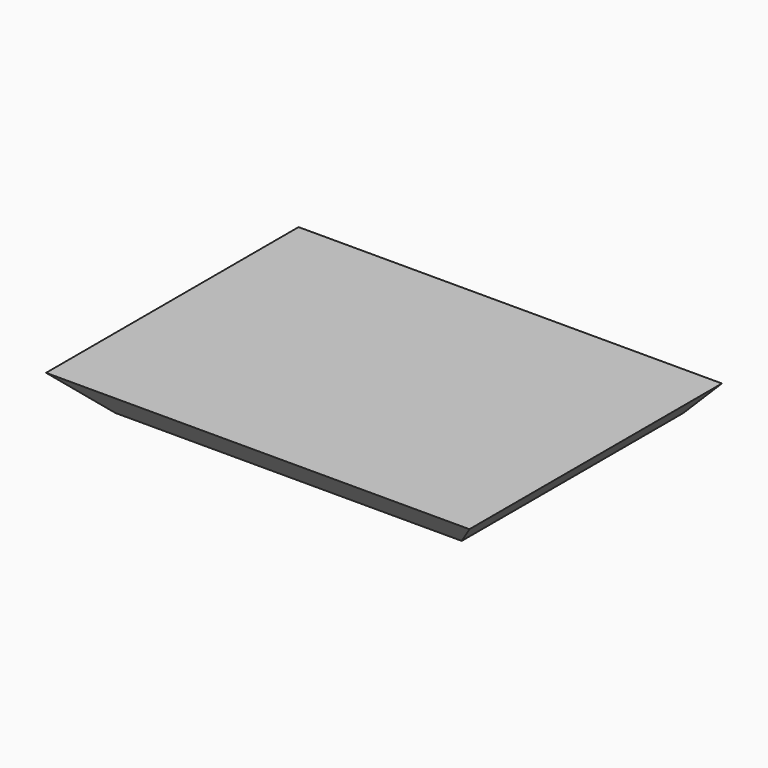
from build123d import *

# Parameters (mm, degrees)
F1_DEPTH = 5
F2_SIZE  = 4.99999


# Not quite as in the source:
# - a fillet or chamfer is up to 0.001 mm smaller than in the source, because OpenCascade refuses the exact size


with BuildPart() as f1:
    # F0 (on Top) → F1 (new body)
    with BuildSketch(Plane.XY):
        Polygon((-27.5, -52.5), (27.5, -52.5), (27.5, -14.74), (-27.5, -11.5), align=None)
        Polygon((-27.5, -11.5), (27.5, -14.74), (27.5, -11.5), align=None)
    extrude(amount=F1_DEPTH)

    # F2 (size 5 in the source; OpenCascade refuses exactly that, so slightly less here)
    f2_edges = [f1.edges().sort_by_distance(p)[0] for p in [
        (-27.5, -32, 0),
        (0, -52.5, 0),
        (27.5, -32, 0),
    ]]
    chamfer(f2_edges, length=F2_SIZE)


solid = f1.part
